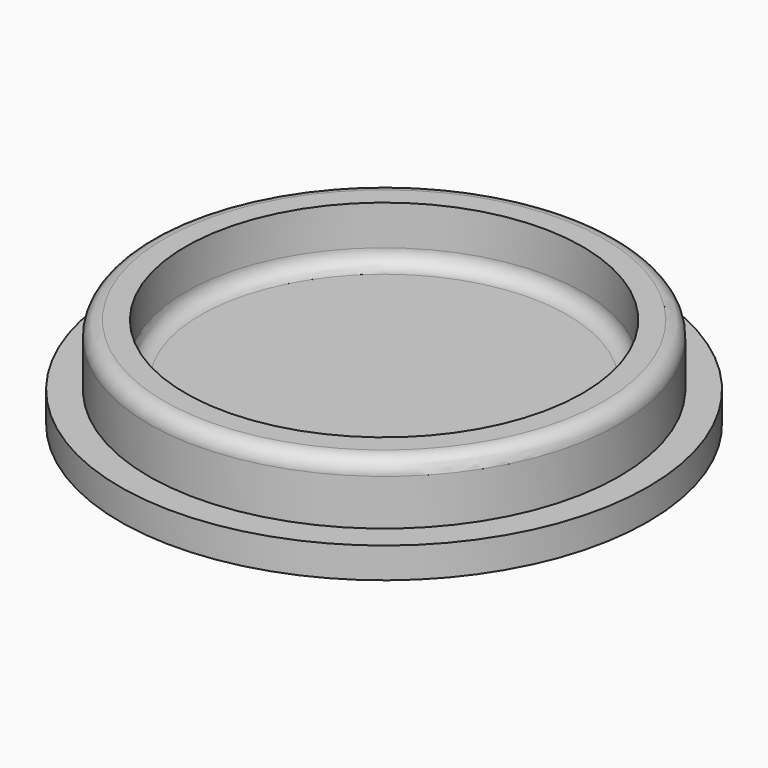
from build123d import *

# Parameters (mm, degrees)
F0_R     = 15.375
F1_DEPTH = 6
F0_R_2   = 17.25
F2_DEPTH = 2
F3_T     = -2.4
F4_R     = 1


with BuildPart() as f1:
    # F0 (on Top) → F1 (new body)
    with BuildSketch(Plane.XY):
        Circle(F0_R)
    extrude(amount=F1_DEPTH)

    # F0 (on Top) → F2 (join)
    with BuildSketch(Plane.XY):
        Circle(F0_R_2)
        Circle(F0_R, mode=Mode.SUBTRACT)
    extrude(amount=F2_DEPTH)

    # F3
    f3_openings = [f1.faces().sort_by_distance(p)[0] for p in [
        (0, 0, 6),
    ]]
    offset(amount=F3_T, openings=f3_openings)

    # F4
    f4_edges = [f1.edges().sort_by_distance(p)[0] for p in [
        (-15.375, 0, 6),
        (-12.975, 0, 2.4),
    ]]
    fillet(f4_edges, radius=F4_R)


solid = f1.part
